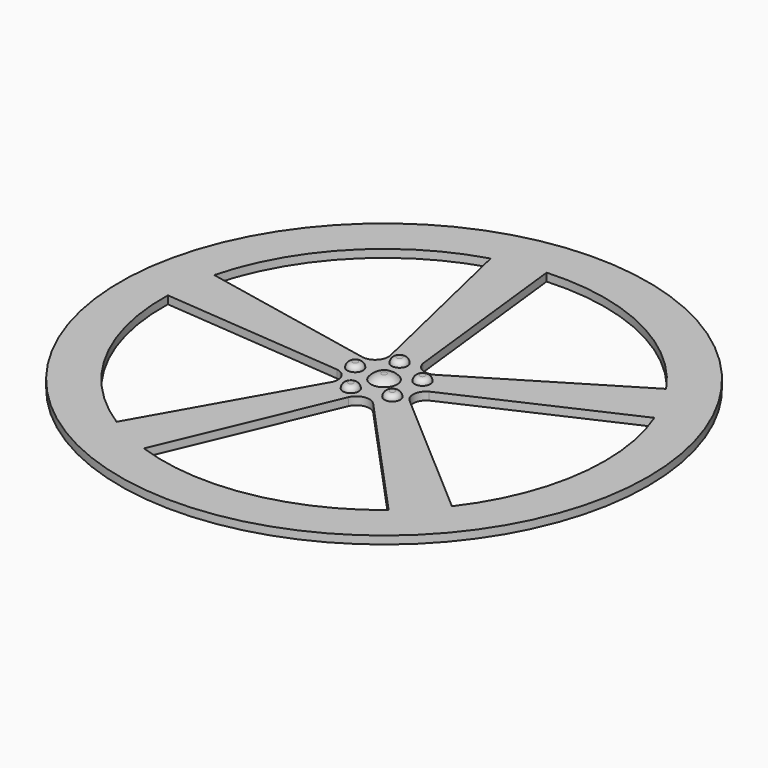
from build123d import *

# Parameters (mm, degrees)
F0_R     = 100
F1_DEPTH = 3
F2_R     = 3
F3_DEPTH = 2
F4_R     = 4.9929816157
F5_DEPTH = 2
F6_R     = 1.99999
F9_DEPTH = 3


# Not quite as in the source:
# - a fillet or chamfer that OpenCascade refuses, or shapes differently, is made with other operations: its cross-section is extruded or revolved along the edge and cut away or added
# - a fillet or chamfer is up to 0.001 mm smaller than in the source, because OpenCascade refuses the exact size


with BuildPart() as f1:
    # F0 (on Top) → F1 (new body)
    with BuildSketch(Plane.XY):
        Circle(F0_R)
    extrude(amount=F1_DEPTH)

    # F2 (on face) → F3 (join)
    with BuildSketch(Plane.XY.offset(3)):
        with Locations((-2.9619428524, 11.0336985157)):
            Circle(F2_R)
        with Locations((9.5783801944, 6.2265754028)):
            Circle(F2_R)
        with Locations((-11.4089615499, 0.5926253015)):
            Circle(F2_R)
        with Locations((-4.0891831618, -10.6674359368)):
            Circle(F2_R)
        with Locations((8.8817073697, -7.1854632832)):
            Circle(F2_R)
    extrude(amount=F3_DEPTH)

    # F4 (on face) → F5 (join)
    with BuildSketch(Plane.XY.offset(3)):
        Circle(F4_R)
    extrude(amount=F5_DEPTH)

    # F6 (radius 2 in the source; OpenCascade refuses exactly that, so slightly less here)
    f6_edges = [f1.edges().sort_by_distance(p)[0] for p in [
        (-5.961943, 11.033699, 5),
        (6.57838, 6.226575, 5),
        (-14.408962, 0.592625, 5),
        (-7.089183, -10.667436, 5),
        (5.881707, -7.185463, 5),
    ]]
    fillet(f6_edges, radius=F6_R)

    # F7: fillet of radius 5 on 1 edges, made by hand

    # F7_s1 → F7_t2 (revolve, cut)
    with BuildSketch(Plane.XZ):
        with BuildLine():
            ThreePointArc((4.9929816157, 3), (3.2290495932, 4.472135955), (0.9929816157, 5))
            Line((0.9929816157, 5), (4.9929816157, 5))
            Line((4.9929816157, 5), (4.9929816157, 3))
        make_face()
    revolve(axis=Axis((0, 0, 5), (0, 0, 1)), mode=Mode.SUBTRACT)

    # F8 (on face) → F9 (cut, through all)
    with BuildSketch(Plane.XY.offset(3)):
        with BuildLine():
            ThreePointArc((66.3999116797, -50.8959301615), (79.2290945271, -26.8718171788), (83.6620820807, 0))
            ThreePointArc((83.6620820807, 0), (82.1834696388, 15.6595432948), (77.7998972031, 30.7655647318))
            Line((77.7998972031, 30.7655647318), (15.2511779268, 2.2686341687))
            Line((15.2511779268, 2.2686341687), (17.7023078517, -2.1256138206))
            Line((17.7023078517, -2.1256138206), (14.2805704694, -5.8146742141))
            Line((14.2805704694, -5.8146742141), (66.3999116797, -50.8959301615))
        make_face()
        with BuildLine():
            Line((9.9430227659, 11.7847964524), (68.923607167, 47.42236132))
            ThreePointArc((68.923607167, 47.42236132), (36.6056794276, 75.2287724991), (-5.2183004193, 83.4991815458))
            Line((-5.2183004193, 83.4991815458), (2.5552738543, 15.2057786606))
            Line((2.5552738543, 15.2057786606), (7.491892841, 16.1790444417))
            Line((7.491892841, 16.1790444417), (9.9430227659, 11.7847964524))
        make_face()
        with BuildLine():
            Line((17.7023078517, -2.1256138206), (15.2511779268, 2.2686341687))
            ThreePointArc((15.2511779268, 2.2686341687), (12.7065485295, -1.5257454222), (14.2805704694, -5.8146742141))
            Line((14.2805704694, -5.8146742141), (17.7023078517, -2.1256138206))
        make_face()
        with BuildLine():
            ThreePointArc((-27.886204899, -78.8777760489), (14.6037462755, -82.3776339354), (53.3012812121, -64.4850168584))
            Line((53.3012812121, -64.4850168584), (6.8704724729, -13.8036856363))
            Line((6.8704724729, -13.8036856363), (3.4487350906, -17.4927460298))
            Line((3.4487350906, -17.4927460298), (-1.1171448371, -15.3784627502))
            Line((-1.1171448371, -15.3784627502), (-27.886204899, -78.8777760489))
        make_face()
        with BuildLine():
            ThreePointArc((2.5552738543, 15.2057786606), (5.3776095614, 11.613164514), (9.9430227659, 11.7847964524))
            Line((9.9430227659, 11.7847964524), (7.491892841, 16.1790444417))
            Line((7.491892841, 16.1790444417), (2.5552738543, 15.2057786606))
        make_face()
        with BuildLine():
            Line((3.4487350906, -17.4927460298), (6.8704724729, -13.8036856363))
            ThreePointArc((6.8704724729, -13.8036856363), (2.4754693095, -12.5561270431), (-1.1171448371, -15.3784627502))
            Line((-1.1171448371, -15.3784627502), (3.4487350906, -17.4927460298))
        make_face()
        with BuildLine():
            Line((-17.7639668564, 54.3390592143), (-23.8027798233, 80.204561284))
            ThreePointArc((-23.8027798233, 80.204561284), (-60.2350372644, 58.0610391212), (-81.0249842257, 20.8397674963))
            Line((-81.0249842257, 20.8397674963), (-55.6504609188, 15.6744066086))
            ThreePointArc((-55.6504609188, 15.6744066086), (-29.7834804383, 28.2223454015), (-17.7639668564, 54.3390592143))
        make_face()
        with BuildLine():
            ThreePointArc((-83.6345341245, 2.1467836063), (-73.8329797706, -39.3450769001), (-44.8578937701, -70.6194969154))
            Line((-44.8578937701, -70.6194969154), (-11.0049924198, -10.799781062))
            Line((-11.0049924198, -10.799781062), (-15.5708723475, -8.6854977824))
            Line((-15.5708723475, -8.6854977824), (-14.971003949, -3.6897384602))
            Line((-14.971003949, -3.6897384602), (-83.6345341245, 2.1467836063))
        make_face()
        with BuildLine():
            Line((-8.1354444491, 13.0980789722), (-17.7639668564, 54.3390592143))
            ThreePointArc((-17.7639668564, 54.3390592143), (-29.7834804383, 28.2223454015), (-55.6504609188, 15.6744066086))
            Line((-55.6504609188, 15.6744066086), (-13.6719318343, 7.1290538689))
            Line((-13.6719318343, 7.1290538689), (-13.0720634358, 12.1248131911))
            Line((-13.0720634358, 12.1248131911), (-8.1354444491, 13.0980789722))
        make_face()
        with BuildLine():
            ThreePointArc((-13.6719318343, 7.1290538689), (-9.3830030423, 8.7030758088), (-8.1354444491, 13.0980789722))
            Line((-8.1354444491, 13.0980789722), (-13.0720634358, 12.1248131911))
            Line((-13.0720634358, 12.1248131911), (-13.6719318343, 7.1290538689))
        make_face()
        with BuildLine():
            Line((-15.5708723475, -8.6854977824), (-11.0049924198, -10.799781062))
            ThreePointArc((-11.0049924198, -10.799781062), (-11.1766243581, -6.2343678575), (-14.971003949, -3.6897384602))
            Line((-14.971003949, -3.6897384602), (-15.5708723475, -8.6854977824))
        make_face()
    extrude(amount=-F9_DEPTH, mode=Mode.SUBTRACT)


solid = f1.part
